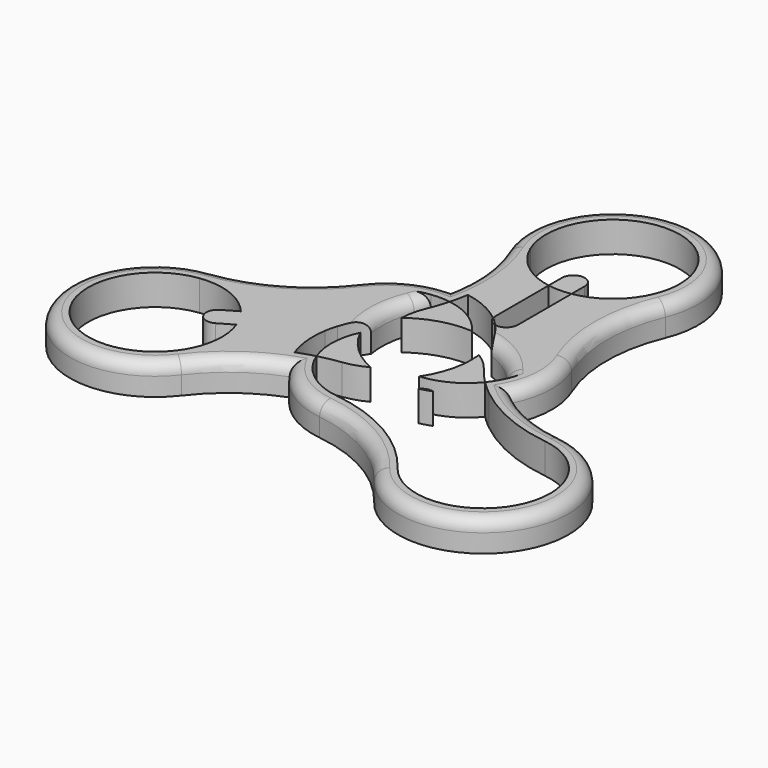
from build123d import *

# Parameters (mm, degrees)
F1_DEPTH     = 5
F2_T3_ANGLE  = 45.2397298961
F2_T6_ANGLE  = 43.7169751844
F2_S7_R      = 14
F2_T8_DEPTH  = 14
F2_T11_ANGLE = 225.2397298961
F2_T14_ANGLE = 43.7169751844
F2_S15_R     = 14
F2_T16_DEPTH = 13
F2_T19_ANGLE = 45.2397298961
F2_T22_ANGLE = 225.2397298961
F2_T25_ANGLE = 45.2397298961
F2_T28_ANGLE = 43.7169751844
F2_S29_R     = 14
F2_T30_DEPTH = 13
F2_T33_ANGLE = 225.2397298961
F2_T36_ANGLE = 53.0691425176
F2_T39_ANGLE = 17.2043081147
F2_S40_R     = 11
F2_T41_DEPTH = 6
F2_T44_ANGLE = 53.0691425176
F2_T47_ANGLE = 17.2043081147
F2_S48_R     = 11
F2_T49_DEPTH = 6
F2_T52_ANGLE = 70.3876536924
F2_S53_R     = 25
F2_T54_DEPTH = 11
F2_T57_ANGLE = 70.3876536924
F2_S58_R     = 25
F2_T59_DEPTH = 11
F2_T62_ANGLE = 70.3876536924
F2_S63_R     = 25
F2_T64_DEPTH = 11
F2_T68_ANGLE = 70.3876536924
F2_S69_R     = 25
F2_T70_DEPTH = 11
F2_T73_ANGLE = 43.7169751844
F2_S74_R     = 14
F2_T75_DEPTH = 14
F2_T80_ANGLE = 43.7169751844
F2_S81_R     = 14
F2_T82_DEPTH = 13
F2_T85_ANGLE = 70.3876536924
F2_S86_R     = 25
F2_T87_DEPTH = 11
F2_T92_ANGLE = 43.7169751844
F2_S93_R     = 14
F2_T94_DEPTH = 13
F2_T97_ANGLE = 70.3876536924
F2_S98_R     = 25
F2_T99_DEPTH = 11


# Not quite as in the source:
# - a fillet or chamfer that OpenCascade refuses, or shapes differently, is made with other operations: its cross-section is extruded or revolved along the edge and cut away or added
# - a feature names something its author has since deleted; it is built from what else it names


with BuildPart() as f1:
    # F0 (on Top) → F1 (new body)
    with BuildSketch(Plane.XY):
        with BuildLine():
            ThreePointArc((-8.9698983934, 7.6942757283), (-9.5052162305, 5.9431554608), (-10.1538461538, 4.2307692308))
            ThreePointArc((-10.1538461538, 4.2307692308), (-10.7496700077, 2.333365536), (-10.994117635, 0.3596907393))
            ThreePointArc((-10.994117635, 0.3596907393), (-6.5804867052, 2.5766497248), (-1.6716579398, 3.1229511789))
            ThreePointArc((-1.6716579398, 3.1229511789), (-4.8548371993, 6.1525005216), (-8.9698983934, 7.6942757283))
        make_face()
    extrude(amount=F1_DEPTH)


with BuildPart() as f1b:
    # F0 (on Top) → F1, piece 2 (new body)
    with BuildSketch(Plane.XY):
        with BuildLine():
            ThreePointArc((-12.0764575971, 7.7429951841), (-10.5214492356, 7.8288685026), (-8.9698983934, 7.6942757283))
            ThreePointArc((-8.9698983934, 7.6942757283), (-8.6169894219, 9.1544263175), (-8.3428968749, 10.6314022012))
            ThreePointArc((-8.3428968749, 10.6314022012), (-9.8429102512, 10.8043309965), (-11.352823103, 10.8147077752))
            ThreePointArc((-11.352823103, 10.8147077752), (-11.6661234513, 9.2674218617), (-12.0764575971, 7.7429951841))
        make_face()
        with BuildLine():
            ThreePointArc((-15.9542013089, -6.6371947227), (-15.0502980655, -4.4401465787), (-13.7879267046, -2.4275661038))
            ThreePointArc((-13.7879267046, -2.4275661038), (-13.9149909666, 1.5404630468), (-12.9230769231, 5.3846153846))
            ThreePointArc((-12.9230769231, 5.3846153846), (-12.4702012833, 6.5531915879), (-12.0764575971, 7.7429951841))
            ThreePointArc((-12.0764575971, 7.7429951841), (-16.1806400059, 6.3641659408), (-19.4348152119, 3.5083250742))
            ThreePointArc((-19.4348152119, 3.5083250742), (-27.6843195603, -3.7415757955), (-38.0876700626, -7.260905695))
            ThreePointArc((-38.0876700626, -7.260905695), (-32.6619159823, -7.9278280654), (-28.2272067116, -11.1242239222))
            Line((-28.2272067116, -11.1242239222), (-18.6734480715, -5.6083587996))
            ThreePointArc((-18.6734480715, -5.6083587996), (-17.0699773971, -5.478280445), (-15.9542013089, -6.6371947227))
        make_face()
        with BuildLine():
            ThreePointArc((-11.352823103, 10.8147077752), (-9.8429102512, 10.8043309965), (-8.3428968749, 10.6314022012))
            ThreePointArc((-8.3428968749, 10.6314022012), (-8.1982358461, 18.3259449677), (-10.1538461538, 25.7692307692))
            ThreePointArc((-10.1538461538, 25.7692307692), (-2.1572774865, 40.7863874326), (11, 30))
            ThreePointArc((11, 30), (10.7863874326, 27.8427225135), (10.1538461538, 25.7692307692))
            ThreePointArc((10.1538461538, 25.7692307692), (8, 15), (10.1538461538, 4.2307692308))
            ThreePointArc((10.1538461538, 4.2307692308), (10.9999892904, -0.0153495993), (10.1419992383, -4.2590904487))
            ThreePointArc((10.1419992383, -4.2590904487), (11.2570243943, -5.3766635818), (12.4403631282, -6.4216325992))
            ThreePointArc((12.4403631282, -6.4216325992), (13.9883128244, -0.5719303522), (12.9230769231, 5.3846153846))
            ThreePointArc((12.9230769231, 5.3846153846), (11, 15), (12.9230769231, 24.6153846154))
            ThreePointArc((12.9230769231, 24.6153846154), (0, 44), (-12.9230769231, 24.6153846154))
            ThreePointArc((-12.9230769231, 24.6153846154), (-11.1602717428, 17.8262873363), (-11.352823103, 10.8147077752))
        make_face()
        with BuildLine():
            ThreePointArc((-10.1538461538, 25.7692307692), (-8.1982358461, 18.3259449677), (-8.3428968749, 10.6314022012))
            ThreePointArc((-8.3428968749, 10.6314022012), (-4.8863165341, 9.5688051601), (-1.8172189569, 7.6562936736))
            ThreePointArc((-1.8172189569, 7.6562936736), (-1.8626550619, 7.8910854725), (-1.8778827507, 8.1297478825))
            Line((-1.8778827507, 8.1297478825), (-1.8778827507, 19.1614781278))
            ThreePointArc((-1.8778827507, 19.1614781278), (-6.8633973986, 21.4038510861), (-10.1538461538, 25.7692307692))
        make_face()
        with BuildLine():
            ThreePointArc((-19.4348152119, 3.5083250742), (-16.1806400059, 6.3641659408), (-12.0764575971, 7.7429951841))
            ThreePointArc((-12.0764575971, 7.7429951841), (-11.6661234513, 9.2674218617), (-11.352823103, 10.8147077752))
            ThreePointArc((-11.352823103, 10.8147077752), (-17.1927887015, 9.2304204123), (-21.8186906778, 5.3296261924))
            ThreePointArc((-21.8186906778, 5.3296261924), (-29.1843195603, -1.1434995841), (-38.4730253659, -4.285758423))
            ThreePointArc((-38.4730253659, -4.285758423), (-48.7990562701, -25.1697790258), (-25.5499484429, -26.6691842439))
            ThreePointArc((-25.5499484429, -26.6691842439), (-20.5518203206, -21.7480015363), (-14.3833386198, -18.4089661252))
            ThreePointArc((-14.3833386198, -18.4089661252), (-15.1293084918, -17.0961548487), (-15.7295544502, -15.7106407612))
            ThreePointArc((-15.7295544502, -15.7106407612), (-22.4655544709, -19.4326320185), (-27.9338239088, -24.8478831257))
            ThreePointArc((-27.9338239088, -24.8478831257), (-46.2009800587, -23.6697790258), (-38.0876700626, -7.260905695))
            ThreePointArc((-38.0876700626, -7.260905695), (-27.6843195603, -3.7415757955), (-19.4348152119, 3.5083250742))
        make_face()
        with BuildLine():
            ThreePointArc((-0.3727386764, 6.2892290685), (1.078009208, 4.4079018251), (2.189769346, 2.3083659201))
            ThreePointArc((2.189769346, 2.3083659201), (5.6897155243, 0.4343922237), (8.5228920831, -2.3467067053))
            ThreePointArc((8.5228920831, -2.3467067053), (9.3084709415, -3.3231966158), (10.1419992383, -4.2590904487))
            ThreePointArc((10.1419992383, -4.2590904487), (10.9999892904, -0.0153495993), (10.1538461538, 4.2307692308))
            ThreePointArc((10.1538461538, 4.2307692308), (8, 15), (10.1538461538, 25.7692307692))
            ThreePointArc((10.1538461538, 25.7692307692), (6.8633973986, 21.4038510861), (1.8778827507, 19.1614781278))
            Line((1.8778827507, 19.1614781278), (1.8778827507, 8.1297478825))
            ThreePointArc((1.8778827507, 8.1297478825), (1.188798573, 6.6760623669), (-0.3727386764, 6.2892290685))
        make_face()
        with BuildLine():
            ThreePointArc((-16.4158738452, -8.5716836435), (-16.2194322852, -7.5962307659), (-15.9542013089, -6.6371947227))
            ThreePointArc((-15.9542013089, -6.6371947227), (-17.0699773971, -5.478280445), (-18.6734480715, -5.6083587996))
            Line((-18.6734480715, -5.6083587996), (-28.2272067116, -11.1242239222))
            ThreePointArc((-28.2272067116, -11.1242239222), (-27.1484211755, -12.6697790258), (-26.3493239609, -14.3768122571))
            Line((-26.3493239609, -14.3768122571), (-16.7955653208, -8.8609471344))
            ThreePointArc((-16.7955653208, -8.8609471344), (-16.5964914552, -8.728428364), (-16.4158738452, -8.5716836435))
        make_face()
        with BuildLine():
            ThreePointArc((-11.3613402358, -17.4997956846), (-12.2132128918, -16.1960555997), (-12.8724275513, -14.7850767679))
            ThreePointArc((-12.8724275513, -14.7850767679), (-14.3134095407, -15.209523928), (-15.7295544502, -15.7106407612))
            ThreePointArc((-15.7295544502, -15.7106407612), (-15.1293084918, -17.0961548487), (-14.3833386198, -18.4089661252))
            ThreePointArc((-14.3833386198, -18.4089661252), (-12.8866995377, -17.9066492291), (-11.3613402358, -17.4997956846))
        make_face()
        with BuildLine():
            ThreePointArc((-15.7295544502, -15.7106407612), (-16.537608589, -12.1858558553), (-16.4158738452, -8.5716836435))
            ThreePointArc((-16.4158738452, -8.5716836435), (-16.5964914552, -8.728428364), (-16.7955653208, -8.8609471344))
            Line((-16.7955653208, -8.8609471344), (-26.3493239609, -14.3768122571))
            ThreePointArc((-26.3493239609, -14.3768122571), (-25.8446696102, -16.2435317958), (-25.6747006171, -18.1697790258))
            ThreePointArc((-25.6747006171, -18.1697790258), (-26.2547763421, -21.6947156357), (-27.9338239088, -24.8478831257))
            ThreePointArc((-27.9338239088, -24.8478831257), (-22.4655544709, -19.4326320185), (-15.7295544502, -15.7106407612))
        make_face()
        with BuildLine():
            ThreePointArc((10.1419992383, -4.2590904487), (9.4388635329, -5.6487038521), (8.54652735, -6.9250899096))
            ThreePointArc((8.54652735, -6.9250899096), (9.6346003679, -7.9607933387), (10.7766527305, -8.9366523893))
            ThreePointArc((10.7766527305, -8.9366523893), (11.6764201484, -7.724067097), (12.4403631282, -6.4216325992))
            ThreePointArc((12.4403631282, -6.4216325992), (11.2570243943, -5.3766635818), (10.1419992383, -4.2590904487))
        make_face()
        with BuildLine():
            ThreePointArc((-4.0148295366, -21.7549852542), (-8.1151478792, -20.3647072907), (-11.3613402358, -17.4997956846))
            ThreePointArc((-11.3613402358, -17.4997956846), (-12.8866995377, -17.9066492291), (-14.3833386198, -18.4089661252))
            ThreePointArc((-14.3833386198, -18.4089661252), (-10.0913227175, -22.6743810093), (-4.4001848399, -24.7301325262))
            ThreePointArc((-4.4001848399, -24.7301325262), (4.8885209657, -27.8723913651), (12.2541498482, -34.3455171416))
            ThreePointArc((12.2541498482, -34.3455171416), (35.5032576754, -32.8461119235), (25.1772267713, -11.9620913207))
            ThreePointArc((25.1772267713, -11.9620913207), (18.4162934687, -10.0941767492), (12.4403631282, -6.4216325992))
            ThreePointArc((12.4403631282, -6.4216325992), (11.6764201484, -7.724067097), (10.7766527305, -8.9366523893))
            ThreePointArc((10.7766527305, -8.9366523893), (17.3679917224, -12.9092038984), (24.791871468, -14.9372385927))
            ThreePointArc((24.791871468, -14.9372385927), (31.6415488109, -18.5846611008), (34.3789020224, -25.8461119235))
            ThreePointArc((34.3789020224, -25.8461119235), (26.9038386324, -36.2660361984), (14.6380253141, -32.5242160234))
            ThreePointArc((14.6380253141, -32.5242160234), (6.3885209657, -25.2743151537), (-4.0148295366, -21.7549852542))
        make_face()
        with BuildLine():
            ThreePointArc((-26.3493239609, -14.3768122571), (-27.1484211755, -12.6697790258), (-28.2272067116, -11.1242239222))
            Line((-28.2272067116, -11.1242239222), (-30.5730737998, -12.4786109171))
            ThreePointArc((-30.5730737998, -12.4786109171), (-31.2604265919, -15.0438464599), (-28.6951910491, -15.7311992519))
            Line((-28.6951910491, -15.7311992519), (-26.3493239609, -14.3768122571))
        make_face()
    extrude(amount=F1_DEPTH)

    # F2: fillet of radius 2 on 16 edges, made by hand


with BuildPart() as f1c:
    # F0 (on Top) → F1, piece 3 (new body)
    with BuildSketch(Plane.XY):
        with BuildLine():
            ThreePointArc((-5.5083810038, -12.8708095595), (-9.6351392692, -10.1569725441), (-12.5626645894, -6.1789528575))
            ThreePointArc((-12.5626645894, -6.1789528575), (-13.5947416524, -10.4504416324), (-12.8724275513, -14.7850767679))
            ThreePointArc((-12.8724275513, -14.7850767679), (-11.0882539959, -14.3731154802), (-9.280969058, -14.0786523565))
            ThreePointArc((-9.280969058, -14.0786523565), (-7.3398573302, -13.6459491028), (-5.5083810038, -12.8708095595))
        make_face()
    extrude(amount=F1_DEPTH)


with BuildPart() as f1d:
    # F0 (on Top) → F1, piece 4 (new body)
    with BuildSketch(Plane.XY):
        with BuildLine():
            ThreePointArc((-0.3727386764, 6.2892290685), (-1.0706727648, 6.9984438534), (-1.8172189569, 7.6562936736))
            ThreePointArc((-1.8172189569, 7.6562936736), (-1.2908117669, 6.7658385718), (-0.3727386764, 6.2892290685))
        make_face()
    extrude(amount=F1_DEPTH)


with BuildPart() as f1e:
    # F0 (on Top) → F1, piece 5 (new body)
    with BuildSketch(Plane.XY):
        with BuildLine():
            ThreePointArc((3.2067000442, -1.504772129), (2.9198273798, -6.4355681298), (0.9385239345, -10.9598892706))
            ThreePointArc((0.9385239345, -10.9598892706), (5.1537802571, -9.7179498384), (8.54652735, -6.9250899096))
            ThreePointArc((8.54652735, -6.9250899096), (7.2976716318, -5.5859309297), (6.1390166172, -4.1680078235))
            ThreePointArc((6.1390166172, -4.1680078235), (4.7937287433, -2.7033073825), (3.2067000442, -1.504772129))
        make_face()
    extrude(amount=F1_DEPTH)


with BuildPart() as f1f:
    # F0 (on Top) → F1, piece 6 (new body)
    with BuildSketch(Plane.XY):
        with BuildLine():
            Line((-1.8778827507, 21.8702521175), (-1.8778827507, 19.1614781278))
            ThreePointArc((-1.8778827507, 19.1614781278), (0, 19), (1.8778827507, 19.1614781278))
            Line((1.8778827507, 19.1614781278), (1.8778827507, 21.8702521175))
            ThreePointArc((1.8778827507, 21.8702521175), (0, 23.7481348682), (-1.8778827507, 21.8702521175))
        make_face()
    extrude(amount=F1_DEPTH)


with BuildPart() as f1g:
    # F0 (on Top) → F1, piece 7 (new body)
    with BuildSketch(Plane.XY):
        with BuildLine():
            ThreePointArc((4.9372942075, -13.1005009793), (3.9029338734, -13.1111554277), (3.0311413907, -13.667925295))
            ThreePointArc((3.0311413907, -13.667925295), (3.9943064553, -13.4181040367), (4.9372942075, -13.1005009793))
        make_face()
    extrude(amount=F1_DEPTH)


with BuildPart() as f2_tool1:
    # F2_s2 → F2_t3 (revolve)
    with BuildSketch(Plane(origin=(0, 0, 0), x_dir=(0, 0, 1), z_dir=(0.3846153846, -0.9230769231, 0))):
        with BuildLine():
            ThreePointArc((3, -14), (4.4142135624, -13.4142135624), (5, -12))
            Line((5, -12), (5, -14))
            Line((5, -14), (3, -14))
        make_face()
    revolve(axis=Axis((36, 15, 5), (0, 0, -1)), revolution_arc=F2_T3_ANGLE)


with BuildPart() as f2_tool4:
    # F2_s5 → F2_t6 (revolve)
    with BuildSketch(Plane(origin=(26.2856287475, -3.4046403465, 0), x_dir=(0, 0, 1), z_dir=(0.9917157573, -0.1284517678, 0))):
        with BuildLine():
            ThreePointArc((3, 8.628935167), (4.4142135624, 9.2147216047), (5, 10.628935167))
            Line((5, 10.628935167), (5, 8.628935167))
            Line((5, 8.628935167), (3, 8.628935167))
        make_face()
    revolve(axis=Axis((28.3885209657, 12.8308026128, 5), (0, 0, -1)), revolution_arc=F2_T6_ANGLE)

    # F2_s7 → F2_t8 (cut, symmetric)
    with BuildSketch(Plane.XY.offset(3.3)):
        Circle(F2_S7_R)
    extrude(amount=F2_T8_DEPTH, both=True, mode=Mode.SUBTRACT)


with BuildPart() as f2_tool9:
    # F2_s10 → F2_t11 (revolve)
    with BuildSketch(Plane(origin=(10.650887574, 25.5621301775, 0), x_dir=(0, 0, 1), z_dir=(-0.3846153846, -0.9230769231, 0))):
        with BuildLine():
            ThreePointArc((3, -2.4615384615), (4.4142135624, -1.8757520239), (5, -0.4615384615))
            Line((5, -0.4615384615), (5, -2.4615384615))
            Line((5, -2.4615384615), (3, -2.4615384615))
        make_face()
    revolve(axis=Axis((0, 30, 5), (0, 0, 1)), revolution_arc=F2_T11_ANGLE)


with BuildPart() as f2_tool12:
    # F2_s13 → F2_t14 (revolve)
    with BuildSketch(Plane(origin=(-10.650887574, 25.5621301775, 0), x_dir=(0, 0, 1), z_dir=(-0.3846153846, 0.9230769231, 0))):
        with BuildLine():
            ThreePointArc((3, -2.4615384615), (4.4142135624, -1.8757520239), (5, -0.4615384615))
            Line((5, -0.4615384615), (5, -2.4615384615))
            Line((5, -2.4615384615), (3, -2.4615384615))
        make_face()
    revolve(axis=Axis((-36, 15, 5), (0, 0, -1)), revolution_arc=F2_T14_ANGLE)

    # F2_s15 → F2_t16 (cut, symmetric)
    with BuildSketch(Plane.XY.offset(4)):
        with Locations((-10.6939385035, -3.1697790258)):
            Circle(F2_S15_R)
    extrude(amount=F2_T16_DEPTH, both=True, mode=Mode.SUBTRACT)


with BuildPart() as f2_tool17:
    # F2_s18 → F2_t19 (revolve)
    with BuildSketch(Plane(origin=(-5.4706301493, -7.160431005, 0), x_dir=(0, 0, 1), z_dir=(0.6071003727, 0.7946251553, 0))):
        with BuildLine():
            ThreePointArc((3, -20.5732985162), (4.4142135624, -19.9875120786), (5, -18.5732985162))
            Line((5, -18.5732985162), (5, -20.5732985162))
            Line((5, -20.5732985162), (3, -20.5732985162))
        make_face()
    revolve(axis=Axis((-41.6843195603, 20.5071355105, 5), (0, 0, -1)), revolution_arc=F2_T19_ANGLE)


with BuildPart() as f2_tool20:
    # F2_s21 → F2_t22 (revolve)
    with BuildSketch(Plane(origin=(-38.3841786231, -4.9717023878, 0), x_dir=(0, 0, 1), z_dir=(0.9917157573, 0.1284517678, 0))):
        with BuildLine():
            ThreePointArc((3, -0.6916739597), (4.4142135624, -0.1058875221), (5, 1.3083260403))
            Line((5, 1.3083260403), (5, -0.6916739597))
            Line((5, -0.6916739597), (3, -0.6916739597))
        make_face()
    revolve(axis=Axis((-36.6747006171, -18.1697790258, 5), (0, 0, 1)), revolution_arc=F2_T22_ANGLE)


with BuildPart() as f2_tool23:
    # F2_s24 → F2_t25 (revolve)
    with BuildSketch(Plane(origin=(-1.177269148, 0.1524855303, 0), x_dir=(0, 0, 1), z_dir=(-0.9917157573, 0.1284517678, 0))):
        with BuildLine():
            ThreePointArc((3, -25.0904736286), (4.4142135624, -24.5046871909), (5, -23.0904736286))
            Line((5, -23.0904736286), (5, -25.0904736286))
            Line((5, -25.0904736286), (3, -25.0904736286))
        make_face()
    revolve(axis=Axis((-7.6114790343, -49.5230264597, 5), (0, 0, -1)), revolution_arc=F2_T25_ANGLE)


with BuildPart() as f2_tool26:
    # F2_s27 → F2_t28 (revolve)
    with BuildSketch(Plane(origin=(-22.2826404709, -29.1654353056, 0), x_dir=(0, 0, 1), z_dir=(-0.6071003727, -0.7946251553, 0))):
        with BuildLine():
            ThreePointArc((3, 4.1117600546), (4.4142135624, 4.6975464923), (5, 6.1117600546))
            Line((5, 6.1117600546), (5, 4.1117600546))
            Line((5, 4.1117600546), (3, 4.1117600546))
        make_face()
    revolve(axis=Axis((-5.6843195603, -41.846693562, 5), (0, 0, -1)), revolution_arc=F2_T28_ANGLE)

    # F2_s29 → F2_t30 (cut, symmetric)
    with BuildSketch(Plane.XY.offset(3.3)):
        with Locations((-2.6018600911, -10.8461119235)):
            Circle(F2_S29_R)
    extrude(amount=F2_T30_DEPTH, both=True, mode=Mode.SUBTRACT)


with BuildPart() as f2_tool31:
    # F2_s32 → F2_t33 (revolve)
    with BuildSketch(Plane(origin=(21.0853917518, -27.5983732644, 0), x_dir=(0, 0, 1), z_dir=(-0.6071003727, 0.7946251553, 0))):
        with BuildLine():
            ThreePointArc((3, -11.1137205318), (4.4142135624, -10.5279340942), (5, -9.1137205318))
            Line((5, -9.1137205318), (5, -11.1137205318))
            Line((5, -11.1137205318), (3, -11.1137205318))
        make_face()
    revolve(axis=Axis((23.3789020224, -25.8461119235, 5), (0, 0, 1)), revolution_arc=F2_T33_ANGLE)


with BuildPart() as f2_tool34:
    # F2_s35 → F2_t36 (revolve)
    with BuildSketch(Plane(origin=(-2.6867450348, -0.0210682014, 0), x_dir=(0, 0, 1), z_dir=(-0.9999692566, -0.0078412925, 0))):
        with BuildLine():
            ThreePointArc((3, 3.174623469), (4.4142135624, 3.7604099066), (5, 5.174623469))
            Line((5, 5.174623469), (5, 3.174623469))
            Line((5, 3.174623469), (3, 3.174623469))
        make_face()
    revolve(axis=Axis((-2.6018600911, -10.8461119235, 5), (0, 0, -1)), revolution_arc=F2_T36_ANGLE)


with BuildPart() as f2_tool37:
    # F2_s38 → F2_t39 (revolve)
    with BuildSketch(Plane(origin=(4.2733814302, -5.5933689637, 0), x_dir=(0, 0, 1), z_dir=(-0.6071003727, 0.7946251553, 0))):
        with BuildLine():
            ThreePointArc((3, 5.3478179297), (4.4142135624, 5.9336043673), (5, 7.3478179297))
            Line((5, 7.3478179297), (5, 5.3478179297))
            Line((5, 5.3478179297), (3, 5.3478179297))
        make_face()
    revolve(axis=Axis((28.3885209657, 12.8308026128, 5), (0, 0, 1)), revolution_arc=F2_T39_ANGLE)

    # F2_s40 → F2_t41 (intersect, symmetric)
    with BuildSketch(Plane.XY.offset(4)):
        Circle(F2_S40_R)
    extrude(amount=F2_T41_DEPTH, both=True, mode=Mode.INTERSECT)


with BuildPart() as f2_tool42:
    # F2_s43 → F2_t44 (revolve)
    with BuildSketch(Plane(origin=(0, 0, 0), x_dir=(0, 0, 1), z_dir=(0.5067753868, -0.862078133, 0))):
        with BuildLine():
            ThreePointArc((3, 14), (4.4142135624, 14.5857864376), (5, 16))
            Line((5, 16), (5, 14))
            Line((5, 14), (3, 14))
        make_face()
    revolve(axis=Axis((0, 0, 5), (0, 0, -1)), revolution_arc=F2_T44_ANGLE)


with BuildPart() as f2_tool45:
    # F2_s46 → F2_t47 (revolve)
    with BuildSketch(Plane(origin=(0, 0, 0), x_dir=(0, 0, 1), z_dir=(-0.3846153846, -0.9230769231, 0))):
        with BuildLine():
            ThreePointArc((3, 14), (4.4142135624, 14.5857864376), (5, 16))
            Line((5, 16), (5, 14))
            Line((5, 14), (3, 14))
        make_face()
    revolve(axis=Axis((-36, 15, 5), (0, 0, 1)), revolution_arc=F2_T47_ANGLE)

    # F2_s48 → F2_t49 (intersect, symmetric)
    with BuildSketch(Plane.XY.offset(4)):
        with Locations((-10.6939385035, -3.1697790258)):
            Circle(F2_S48_R)
    extrude(amount=F2_T49_DEPTH, both=True, mode=Mode.INTERSECT)


with BuildPart() as f2_tool50:
    # F2_s51 → F2_t52 (revolve)
    with BuildSketch(Plane(origin=(0, 0, 0), x_dir=(0, 0, 1), z_dir=(-0.740426843, -0.6721369579, 0))):
        with BuildLine():
            ThreePointArc((3, -14), (4.4142135624, -13.4142135624), (5, -12))
            Line((5, -12), (5, -14))
            Line((5, -14), (3, -14))
        make_face()
    revolve(axis=Axis((0, 0, 5), (0, 0, 1)), revolution_arc=F2_T52_ANGLE)

    # F2_s53 → F2_t54 (intersect, symmetric)
    with BuildSketch(Plane.XY.offset(4)):
        with Locations((28.3885209657, 12.8308026128)):
            Circle(F2_S53_R)
    extrude(amount=F2_T54_DEPTH, both=True, mode=Mode.INTERSECT)


with BuildPart() as f2_tool55:
    # F2_s56 → F2_t57 (revolve)
    with BuildSketch(Plane(origin=(-8.776939983, 2.8125251515, 0), x_dir=(0, 0, 1), z_dir=(0.9523011019, -0.3051599767, 0))):
        with BuildLine():
            ThreePointArc((3, -7.7180539164), (4.4142135624, -7.1322674788), (5, -5.7180539164))
            Line((5, -5.7180539164), (5, -7.7180539164))
            Line((5, -7.7180539164), (3, -7.7180539164))
        make_face()
    revolve(axis=Axis((-10.6939385035, -3.1697790258, 5), (0, 0, 1)), revolution_arc=F2_T57_ANGLE)

    # F2_s58 → F2_t59 (intersect, symmetric)
    with BuildSketch(Plane.XY.offset(4)):
        with Locations((-36, 15)):
            Circle(F2_S58_R)
    extrude(amount=F2_T59_DEPTH, both=True, mode=Mode.INTERSECT)


with BuildPart() as f2_tool60:
    # F2_s61 → F2_t62 (revolve)
    with BuildSketch(Plane(origin=(2.1290406857, -9.8204706261, 0), x_dir=(0, 0, 1), z_dir=(-0.2118742589, 0.9772969346, 0))):
        with BuildLine():
            ThreePointArc((3, -18.8408018169), (4.4142135624, -18.2550153793), (5, -16.8408018169))
            Line((5, -16.8408018169), (5, -18.8408018169))
            Line((5, -18.8408018169), (3, -18.8408018169))
        make_face()
    revolve(axis=Axis((-2.6018600911, -10.8461119235, 5), (0, 0, 1)), revolution_arc=F2_T62_ANGLE)

    # F2_s63 → F2_t64 (intersect, symmetric)
    with BuildSketch(Plane.XY.offset(4)):
        with Locations((-5.6843195603, -41.846693562)):
            Circle(F2_S63_R)
    extrude(amount=F2_T64_DEPTH, both=True, mode=Mode.INTERSECT)


with BuildPart() as f2_tool66:
    # F2_s67 → F2_t68 (revolve)
    with BuildSketch(Plane(origin=(0, 0, 0), x_dir=(0, 0, 1), z_dir=(-0.740426843, -0.6721369579, 0))):
        with BuildLine():
            ThreePointArc((3, -14), (4.4142135624, -13.4142135624), (5, -12))
            Line((5, -12), (5, -14))
            Line((5, -14), (3, -14))
        make_face()
    revolve(axis=Axis((0, 0, 5), (0, 0, 1)), revolution_arc=F2_T68_ANGLE)

    # F2_s69 → F2_t70 (cut, symmetric)
    with BuildSketch(Plane.XY.offset(4)):
        with Locations((28.3885209657, 12.8308026128)):
            Circle(F2_S69_R)
    extrude(amount=F2_T70_DEPTH, both=True, mode=Mode.SUBTRACT)


with BuildPart() as f2_tool71:
    # F2_s72 → F2_t73 (revolve)
    with BuildSketch(Plane(origin=(26.2856287475, -3.4046403465, 0), x_dir=(0, 0, 1), z_dir=(0.9917157573, -0.1284517678, 0))):
        with BuildLine():
            ThreePointArc((3, 8.628935167), (4.4142135624, 9.2147216047), (5, 10.628935167))
            Line((5, 10.628935167), (5, 8.628935167))
            Line((5, 8.628935167), (3, 8.628935167))
        make_face()
    revolve(axis=Axis((28.3885209657, 12.8308026128, 5), (0, 0, -1)), revolution_arc=F2_T73_ANGLE)

    # F2_s74 → F2_t75 (intersect, symmetric)
    with BuildSketch(Plane.XY.offset(3.3)):
        Circle(F2_S74_R)
    extrude(amount=F2_T75_DEPTH, both=True, mode=Mode.INTERSECT)


with BuildPart() as f2_tool66_1:
    add(f2_tool66.part)

    # F2_t76: intersect F2_tool71
    add(f2_tool71.part, mode=Mode.INTERSECT)


with BuildPart() as f2_tool78:
    # F2_s79 → F2_t80 (revolve)
    with BuildSketch(Plane(origin=(-10.650887574, 25.5621301775, 0), x_dir=(0, 0, 1), z_dir=(-0.3846153846, 0.9230769231, 0))):
        with BuildLine():
            ThreePointArc((3, -2.4615384615), (4.4142135624, -1.8757520239), (5, -0.4615384615))
            Line((5, -0.4615384615), (5, -2.4615384615))
            Line((5, -2.4615384615), (3, -2.4615384615))
        make_face()
    revolve(axis=Axis((-36, 15, 5), (0, 0, -1)), revolution_arc=F2_T80_ANGLE)

    # F2_s81 → F2_t82 (intersect, symmetric)
    with BuildSketch(Plane.XY.offset(4)):
        with Locations((-10.6939385035, -3.1697790258)):
            Circle(F2_S81_R)
    extrude(amount=F2_T82_DEPTH, both=True, mode=Mode.INTERSECT)


with BuildPart() as f2_tool83:
    # F2_s84 → F2_t85 (revolve)
    with BuildSketch(Plane(origin=(-8.776939983, 2.8125251515, 0), x_dir=(0, 0, 1), z_dir=(0.9523011019, -0.3051599767, 0))):
        with BuildLine():
            ThreePointArc((3, -7.7180539164), (4.4142135624, -7.1322674788), (5, -5.7180539164))
            Line((5, -5.7180539164), (5, -7.7180539164))
            Line((5, -7.7180539164), (3, -7.7180539164))
        make_face()
    revolve(axis=Axis((-10.6939385035, -3.1697790258, 5), (0, 0, 1)), revolution_arc=F2_T85_ANGLE)

    # F2_s86 → F2_t87 (cut, symmetric)
    with BuildSketch(Plane.XY.offset(4)):
        with Locations((-36, 15)):
            Circle(F2_S86_R)
    extrude(amount=F2_T87_DEPTH, both=True, mode=Mode.SUBTRACT)


with BuildPart() as f2_tool78_1:
    add(f2_tool78.part)

    # F2_t88: intersect F2_tool83
    add(f2_tool83.part, mode=Mode.INTERSECT)


with BuildPart() as f2_tool90:
    # F2_s91 → F2_t92 (revolve)
    with BuildSketch(Plane(origin=(-22.2826404709, -29.1654353056, 0), x_dir=(0, 0, 1), z_dir=(-0.6071003727, -0.7946251553, 0))):
        with BuildLine():
            ThreePointArc((3, 4.1117600546), (4.4142135624, 4.6975464923), (5, 6.1117600546))
            Line((5, 6.1117600546), (5, 4.1117600546))
            Line((5, 4.1117600546), (3, 4.1117600546))
        make_face()
    revolve(axis=Axis((-5.6843195603, -41.846693562, 5), (0, 0, -1)), revolution_arc=F2_T92_ANGLE)

    # F2_s93 → F2_t94 (intersect, symmetric)
    with BuildSketch(Plane.XY.offset(3.3)):
        with Locations((-2.6018600911, -10.8461119235)):
            Circle(F2_S93_R)
    extrude(amount=F2_T94_DEPTH, both=True, mode=Mode.INTERSECT)


with BuildPart() as f2_tool95:
    # F2_s96 → F2_t97 (revolve)
    with BuildSketch(Plane(origin=(2.1290406857, -9.8204706261, 0), x_dir=(0, 0, 1), z_dir=(-0.2118742589, 0.9772969346, 0))):
        with BuildLine():
            ThreePointArc((3, -18.8408018169), (4.4142135624, -18.2550153793), (5, -16.8408018169))
            Line((5, -16.8408018169), (5, -18.8408018169))
            Line((5, -18.8408018169), (3, -18.8408018169))
        make_face()
    revolve(axis=Axis((-2.6018600911, -10.8461119235, 5), (0, 0, 1)), revolution_arc=F2_T97_ANGLE)

    # F2_s98 → F2_t99 (cut, symmetric)
    with BuildSketch(Plane.XY.offset(4)):
        with Locations((-5.6843195603, -41.846693562)):
            Circle(F2_S98_R)
    extrude(amount=F2_T99_DEPTH, both=True, mode=Mode.SUBTRACT)


with BuildPart() as f2_tool90_1:
    add(f2_tool90.part)

    # F2_t100: intersect F2_tool95
    add(f2_tool95.part, mode=Mode.INTERSECT)


with BuildPart() as f1b_1:
    add(f1b.part)

    # F2_t101: cut F2_tool1, F2_tool4, F2_tool9, F2_tool12, F2_tool17, F2_tool20, F2_tool23, F2_tool26, F2_tool31, F2_tool34, F2_tool37, F2_tool42, F2_tool45, F2_tool50, F2_tool55, F2_tool60, F2_tool66, F2_tool78, F2_tool90
    add([f2_tool1.part, f2_tool4.part, f2_tool9.part, f2_tool12.part, f2_tool17.part, f2_tool20.part, f2_tool23.part, f2_tool26.part, f2_tool31.part, f2_tool34.part, f2_tool37.part, f2_tool42.part, f2_tool45.part, f2_tool50.part, f2_tool55.part, f2_tool60.part, f2_tool66_1.part, f2_tool78_1.part, f2_tool90_1.part], mode=Mode.SUBTRACT)


solid = Compound([f1.part, f1c.part, f1d.part, f1e.part, f1f.part, f1g.part, f1b_1.part])
